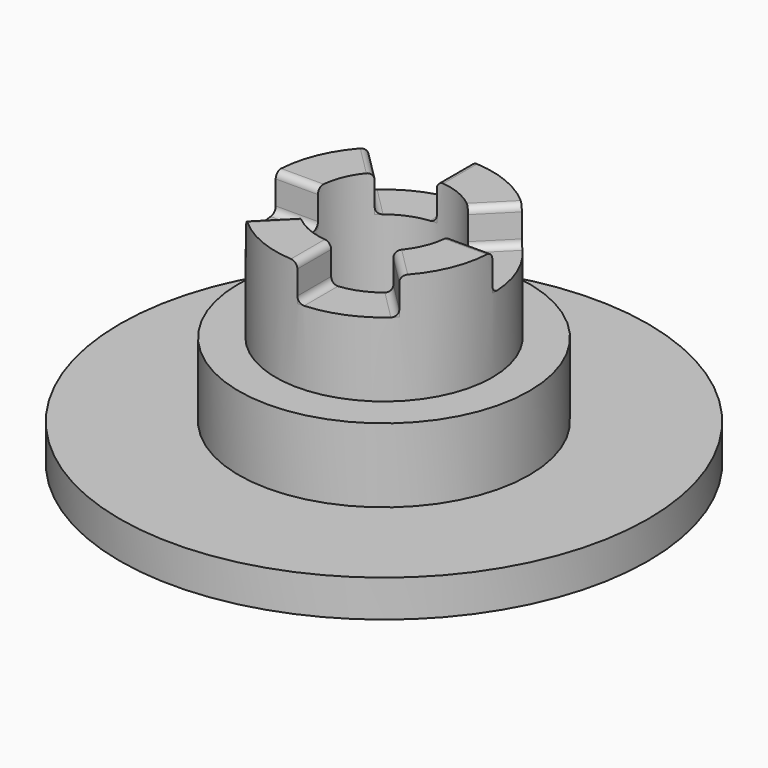
from build123d import *

# Parameters (mm, degrees)
F0_R         = 10
F1_DEPTH     = 1.4
F2_R         = 5.5
F3_DEPTH     = 2.8
F4_R         = 4.1
F4_R_2       = 2.5
F5_DEPTH     = 4.2
F7_DEPTH     = 1.4
F8_T4_DEPTH  = 2.85
F8_S5_R      = 4.1
F8_T6_DEPTH  = 3
F8_S7_R      = 2.5
F8_T8_DEPTH  = 3
F8_T12_DEPTH = 2.85
F8_S13_R     = 4.1
F8_T14_DEPTH = 3
F8_S15_R     = 2.5
F8_T16_DEPTH = 3
F8_T20_DEPTH = 2.85
F8_S21_R     = 4.1
F8_T22_DEPTH = 3
F8_S23_R     = 2.5
F8_T24_DEPTH = 3
F8_T28_DEPTH = 2.85
F8_S29_R     = 4.1
F8_T30_DEPTH = 3
F8_S31_R     = 2.5
F8_T32_DEPTH = 3
F8_T36_DEPTH = 2.85
F8_S37_R     = 4.1
F8_T38_DEPTH = 3
F8_S39_R     = 2.5
F8_T40_DEPTH = 3
F8_T44_DEPTH = 2.85
F8_S45_R     = 4.1
F8_T46_DEPTH = 3
F8_S47_R     = 2.5
F8_T48_DEPTH = 3
F8_T52_DEPTH = 2.85
F8_S53_R     = 4.1
F8_T54_DEPTH = 3
F8_S55_R     = 2.5
F8_T56_DEPTH = 3
F8_T60_DEPTH = 2.85
F8_S61_R     = 4.1
F8_T62_DEPTH = 3
F8_S63_R     = 2.5
F8_T64_DEPTH = 3
F8_T65_DEPTH = 2.85
F8_T67_DEPTH = 2.85
F8_T69_DEPTH = 2.85
F8_T71_DEPTH = 2.85
F8_T73_DEPTH = 2.85
F8_T75_DEPTH = 2.85
F8_T77_DEPTH = 2.85
F8_T79_DEPTH = 2.85


# Not quite as in the source:
# - a fillet or chamfer that OpenCascade refuses, or shapes differently, is made with other operations: its cross-section is extruded or revolved along the edge and cut away or added


with BuildPart() as f1:
    # F0 (on Top) → F1 (new body)
    with BuildSketch(Plane.XY):
        Circle(F0_R)
    extrude(amount=F1_DEPTH)

    # F2 (on face) → F3 (join)
    with BuildSketch(Plane.XY.offset(1.4)):
        Circle(F2_R)
    extrude(amount=F3_DEPTH)

    # F4 (on face) → F5 (join)
    with BuildSketch(Plane.XY.offset(4.2)):
        Circle(F4_R)
        Circle(F4_R_2, mode=Mode.SUBTRACT)
    extrude(amount=F5_DEPTH)

    # F6 (on face) → F7 (cut)
    with BuildSketch(Plane.XY.offset(8.4)):
        with BuildLine():
            Line((0, -2.5), (0, -4.1))
            ThreePointArc((0, -4.1), (1.5690020727, -3.7879060833), (2.8991378029, -2.8991378029))
            Line((2.8991378029, -2.8991378029), (1.767766953, -1.767766953))
            ThreePointArc((1.767766953, -1.767766953), (0.9567085809, -2.3096988313), (0, -2.5))
        make_face()
        with BuildLine():
            ThreePointArc((-4.1, 0), (-3.7879060833, -1.5690020727), (-2.8991378029, -2.8991378029))
            Line((-2.8991378029, -2.8991378029), (-1.767766953, -1.767766953))
            ThreePointArc((-1.767766953, -1.767766953), (-2.3096988313, -0.9567085809), (-2.5, 0))
            Line((-2.5, 0), (-4.1, 0))
        make_face()
        with BuildLine():
            Line((2.5, 0), (4.1, 0))
            ThreePointArc((4.1, 0), (3.7879060833, 1.5690020727), (2.8991378029, 2.8991378029))
            Line((2.8991378029, 2.8991378029), (1.767766953, 1.767766953))
            ThreePointArc((1.767766953, 1.767766953), (2.3096988313, 0.9567085809), (2.5, 0))
        make_face()
        with BuildLine():
            ThreePointArc((-1.767766953, 1.767766953), (-0.9567085809, 2.3096988313), (0, 2.5))
            Line((0, 2.5), (0, 4.1))
            ThreePointArc((0, 4.1), (-1.5690020727, 3.7879060833), (-2.8991378029, 2.8991378029))
            Line((-2.8991378029, 2.8991378029), (-1.767766953, 1.767766953))
        make_face()
    extrude(amount=-F7_DEPTH, mode=Mode.SUBTRACT)

    # F8: fillet of radius 0.25 on 16 edges, made by hand


with BuildPart() as f8_tool2:
    # F8_s3 → F8_t4 (new body)
    with BuildSketch(Plane.YZ.offset(-1.875)):
        with BuildLine():
            ThreePointArc((-0.25, 7), (-0.0732233047, 7.0732233047), (0, 7.25))
            Line((0, 7.25), (0, 7))
            Line((0, 7), (-0.25, 7))
        make_face()
    extrude(amount=-F8_T4_DEPTH)

    # F8_s5 → F8_t6 (intersect, symmetric)
    with BuildSketch(Plane.XY.offset(7.1)):
        Circle(F8_S5_R)
    extrude(amount=F8_T6_DEPTH, both=True, mode=Mode.INTERSECT)

    # F8_s7 → F8_t8 (cut, symmetric)
    with BuildSketch(Plane.XY.offset(7.1)):
        Circle(F8_S7_R)
    extrude(amount=F8_T8_DEPTH, both=True, mode=Mode.SUBTRACT)


with BuildPart() as f1_1:
    add(f1.part)

    # F8_t1: union F8_tool2
    add(f8_tool2.part)


with BuildPart() as f8_tool10:
    # F8_s11 → F8_t12 (new body)
    with BuildSketch(Plane.XZ.offset(-1.875)):
        with BuildLine():
            ThreePointArc((-0.25, 7), (-0.0732233047, 7.0732233047), (0, 7.25))
            Line((0, 7.25), (0, 7))
            Line((0, 7), (-0.25, 7))
        make_face()
    extrude(amount=-F8_T12_DEPTH)

    # F8_s13 → F8_t14 (intersect, symmetric)
    with BuildSketch(Plane.XY.offset(7.1)):
        Circle(F8_S13_R)
    extrude(amount=F8_T14_DEPTH, both=True, mode=Mode.INTERSECT)

    # F8_s15 → F8_t16 (cut, symmetric)
    with BuildSketch(Plane.XY.offset(7.1)):
        Circle(F8_S15_R)
    extrude(amount=F8_T16_DEPTH, both=True, mode=Mode.SUBTRACT)


with BuildPart() as f1_2:
    add(f1_1.part)

    # F8_t9: union F8_tool10
    add(f8_tool10.part)


with BuildPart() as f8_tool18:
    # F8_s19 → F8_t20 (new body)
    with BuildSketch(Plane(origin=(3.3410795411, -3.3410795411, 0), x_dir=(0, 0, 1), z_dir=(-0.7071067812, 0.7071067812, 0))):
        with BuildLine():
            ThreePointArc((7.25, 0), (7.0732233047, -0.0732233047), (7, -0.25))
            Line((7, -0.25), (7, 0))
            Line((7, 0), (7.25, 0))
        make_face()
    extrude(amount=F8_T20_DEPTH)

    # F8_s21 → F8_t22 (intersect, symmetric)
    with BuildSketch(Plane.XY.offset(7.1)):
        Circle(F8_S21_R)
    extrude(amount=F8_T22_DEPTH, both=True, mode=Mode.INTERSECT)

    # F8_s23 → F8_t24 (cut, symmetric)
    with BuildSketch(Plane.XY.offset(7.1)):
        Circle(F8_S23_R)
    extrude(amount=F8_T24_DEPTH, both=True, mode=Mode.SUBTRACT)


with BuildPart() as f1_3:
    add(f1_2.part)

    # F8_t17: union F8_tool18
    add(f8_tool18.part)


with BuildPart() as f8_tool26:
    # F8_s27 → F8_t28 (new body)
    with BuildSketch(Plane.YZ.offset(1.875)):
        with BuildLine():
            ThreePointArc((0, 7.25), (0.0732233047, 7.0732233047), (0.25, 7))
            Line((0.25, 7), (0, 7))
            Line((0, 7), (0, 7.25))
        make_face()
    extrude(amount=F8_T28_DEPTH)

    # F8_s29 → F8_t30 (intersect, symmetric)
    with BuildSketch(Plane.XY.offset(7.1)):
        Circle(F8_S29_R)
    extrude(amount=F8_T30_DEPTH, both=True, mode=Mode.INTERSECT)

    # F8_s31 → F8_t32 (cut, symmetric)
    with BuildSketch(Plane.XY.offset(7.1)):
        Circle(F8_S31_R)
    extrude(amount=F8_T32_DEPTH, both=True, mode=Mode.SUBTRACT)


with BuildPart() as f1_4:
    add(f1_3.part)

    # F8_t25: union F8_tool26
    add(f8_tool26.part)


with BuildPart() as f8_tool34:
    # F8_s35 → F8_t36 (new body)
    with BuildSketch(Plane(origin=(-3.3410795411, -3.3410795411, 0), x_dir=(0, 0, 1), z_dir=(0.7071067812, 0.7071067812, 0))):
        with BuildLine():
            ThreePointArc((7.25, 0), (7.0732233047, -0.0732233047), (7, -0.25))
            Line((7, -0.25), (7, 0))
            Line((7, 0), (7.25, 0))
        make_face()
    extrude(amount=F8_T36_DEPTH)

    # F8_s37 → F8_t38 (intersect, symmetric)
    with BuildSketch(Plane.XY.offset(7.1)):
        Circle(F8_S37_R)
    extrude(amount=F8_T38_DEPTH, both=True, mode=Mode.INTERSECT)

    # F8_s39 → F8_t40 (cut, symmetric)
    with BuildSketch(Plane.XY.offset(7.1)):
        Circle(F8_S39_R)
    extrude(amount=F8_T40_DEPTH, both=True, mode=Mode.SUBTRACT)


with BuildPart() as f1_5:
    add(f1_4.part)

    # F8_t33: union F8_tool34
    add(f8_tool34.part)


with BuildPart() as f8_tool42:
    # F8_s43 → F8_t44 (new body)
    with BuildSketch(Plane(origin=(-3.3410795411, 3.3410795411, 0), x_dir=(0, 0, 1), z_dir=(0.7071067812, -0.7071067812, 0))):
        with BuildLine():
            ThreePointArc((7.25, 0), (7.0732233047, -0.0732233047), (7, -0.25))
            Line((7, -0.25), (7, 0))
            Line((7, 0), (7.25, 0))
        make_face()
    extrude(amount=F8_T44_DEPTH)

    # F8_s45 → F8_t46 (intersect, symmetric)
    with BuildSketch(Plane.XY.offset(7.1)):
        Circle(F8_S45_R)
    extrude(amount=F8_T46_DEPTH, both=True, mode=Mode.INTERSECT)

    # F8_s47 → F8_t48 (cut, symmetric)
    with BuildSketch(Plane.XY.offset(7.1)):
        Circle(F8_S47_R)
    extrude(amount=F8_T48_DEPTH, both=True, mode=Mode.SUBTRACT)


with BuildPart() as f1_6:
    add(f1_5.part)

    # F8_t41: union F8_tool42
    add(f8_tool42.part)


with BuildPart() as f8_tool50:
    # F8_s51 → F8_t52 (new body)
    with BuildSketch(Plane.XZ.offset(1.875)):
        with BuildLine():
            ThreePointArc((0.25, 7), (0.0732233047, 7.0732233047), (0, 7.25))
            Line((0, 7.25), (0, 7))
            Line((0, 7), (0.25, 7))
        make_face()
    extrude(amount=F8_T52_DEPTH)

    # F8_s53 → F8_t54 (intersect, symmetric)
    with BuildSketch(Plane.XY.offset(7.1)):
        Circle(F8_S53_R)
    extrude(amount=F8_T54_DEPTH, both=True, mode=Mode.INTERSECT)

    # F8_s55 → F8_t56 (cut, symmetric)
    with BuildSketch(Plane.XY.offset(7.1)):
        Circle(F8_S55_R)
    extrude(amount=F8_T56_DEPTH, both=True, mode=Mode.SUBTRACT)


with BuildPart() as f1_7:
    add(f1_6.part)

    # F8_t49: union F8_tool50
    add(f8_tool50.part)


with BuildPart() as f8_tool58:
    # F8_s59 → F8_t60 (new body)
    with BuildSketch(Plane(origin=(3.3410795411, 3.3410795411, 0), x_dir=(0, 0, 1), z_dir=(-0.7071067812, -0.7071067812, 0))):
        with BuildLine():
            ThreePointArc((7.25, 0), (7.0732233047, -0.0732233047), (7, -0.25))
            Line((7, -0.25), (7, 0))
            Line((7, 0), (7.25, 0))
        make_face()
    extrude(amount=F8_T60_DEPTH)

    # F8_s61 → F8_t62 (intersect, symmetric)
    with BuildSketch(Plane.XY.offset(7.1)):
        Circle(F8_S61_R)
    extrude(amount=F8_T62_DEPTH, both=True, mode=Mode.INTERSECT)

    # F8_s63 → F8_t64 (cut, symmetric)
    with BuildSketch(Plane.XY.offset(7.1)):
        Circle(F8_S63_R)
    extrude(amount=F8_T64_DEPTH, both=True, mode=Mode.SUBTRACT)


with BuildPart() as f1_8:
    add(f1_7.part)

    # F8_t57: union F8_tool58
    add(f8_tool58.part)

    # F8_s66 → F8_t65 (cut)
    with BuildSketch(Plane.YZ.offset(-4.725)):
        with BuildLine():
            ThreePointArc((0, 8.15), (0.0732233047, 8.3267766953), (0.25, 8.4))
            Line((0.25, 8.4), (0, 8.4))
            Line((0, 8.4), (0, 8.15))
        make_face()
    extrude(amount=F8_T65_DEPTH, mode=Mode.SUBTRACT)

    # F8_s68 → F8_t67 (cut)
    with BuildSketch(Plane(origin=(-3.3410795411, 3.3410795411, 0), x_dir=(0, 0, 1), z_dir=(0.7071067812, -0.7071067812, 0))):
        with BuildLine():
            ThreePointArc((8.4, 0.25), (8.3267766953, 0.0732233047), (8.15, 0))
            Line((8.15, 0), (8.4, 0))
            Line((8.4, 0), (8.4, 0.25))
        make_face()
    extrude(amount=F8_T67_DEPTH, mode=Mode.SUBTRACT)

    # F8_s70 → F8_t69 (cut)
    with BuildSketch(Plane.XZ.offset(1.875)):
        with BuildLine():
            ThreePointArc((0, 8.15), (-0.0732233047, 8.3267766953), (-0.25, 8.4))
            Line((-0.25, 8.4), (0, 8.4))
            Line((0, 8.4), (0, 8.15))
        make_face()
    extrude(amount=F8_T69_DEPTH, mode=Mode.SUBTRACT)

    # F8_s72 → F8_t71 (cut)
    with BuildSketch(Plane(origin=(-3.3410795411, -3.3410795411, 0), x_dir=(0, 0, 1), z_dir=(0.7071067812, 0.7071067812, 0))):
        with BuildLine():
            ThreePointArc((8.4, 0.25), (8.3267766953, 0.0732233047), (8.15, 0))
            Line((8.15, 0), (8.4, 0))
            Line((8.4, 0), (8.4, 0.25))
        make_face()
    extrude(amount=F8_T71_DEPTH, mode=Mode.SUBTRACT)

    # F8_s74 → F8_t73 (cut)
    with BuildSketch(Plane.YZ.offset(1.875)):
        with BuildLine():
            ThreePointArc((0, 8.15), (-0.0732233047, 8.3267766953), (-0.25, 8.4))
            Line((-0.25, 8.4), (0, 8.4))
            Line((0, 8.4), (0, 8.15))
        make_face()
    extrude(amount=F8_T73_DEPTH, mode=Mode.SUBTRACT)

    # F8_s76 → F8_t75 (cut)
    with BuildSketch(Plane(origin=(3.3410795411, -3.3410795411, 0), x_dir=(0, 0, 1), z_dir=(-0.7071067812, 0.7071067812, 0))):
        with BuildLine():
            ThreePointArc((8.4, 0.25), (8.3267766953, 0.0732233047), (8.15, 0))
            Line((8.15, 0), (8.4, 0))
            Line((8.4, 0), (8.4, 0.25))
        make_face()
    extrude(amount=F8_T75_DEPTH, mode=Mode.SUBTRACT)

    # F8_s78 → F8_t77 (cut)
    with BuildSketch(Plane.XZ.offset(-4.725)):
        with BuildLine():
            ThreePointArc((0, 8.15), (0.0732233047, 8.3267766953), (0.25, 8.4))
            Line((0.25, 8.4), (0, 8.4))
            Line((0, 8.4), (0, 8.15))
        make_face()
    extrude(amount=F8_T77_DEPTH, mode=Mode.SUBTRACT)

    # F8_s80 → F8_t79 (cut)
    with BuildSketch(Plane(origin=(3.3410795411, 3.3410795411, 0), x_dir=(0, 0, 1), z_dir=(-0.7071067812, -0.7071067812, 0))):
        with BuildLine():
            ThreePointArc((8.4, 0.25), (8.3267766953, 0.0732233047), (8.15, 0))
            Line((8.15, 0), (8.4, 0))
            Line((8.4, 0), (8.4, 0.25))
        make_face()
    extrude(amount=F8_T79_DEPTH, mode=Mode.SUBTRACT)


solid = f1_8.part
